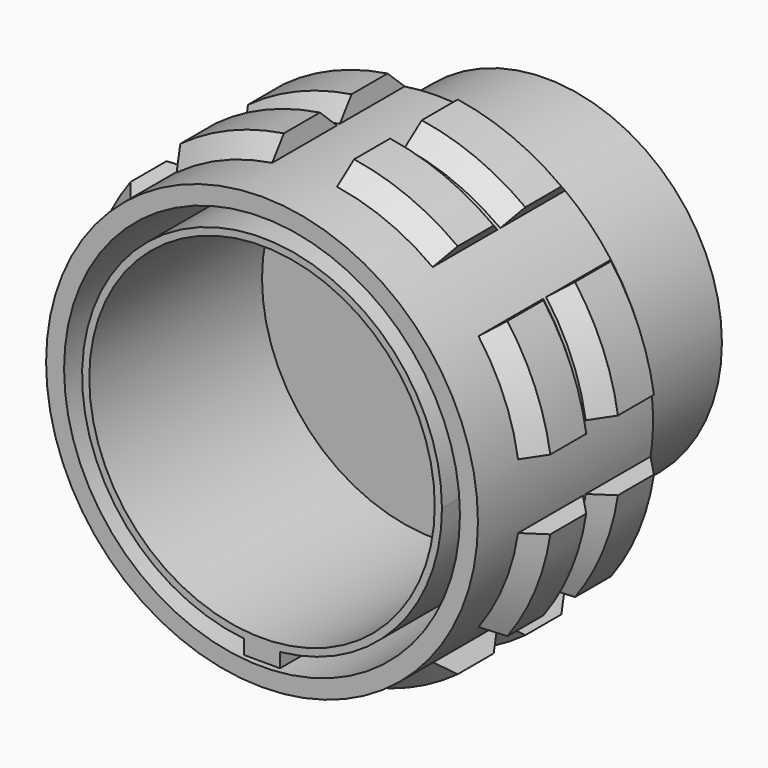
from build123d import *

# Parameters (mm, degrees)
F0_R      = 19.05
F1_DEPTH  = 15.6718
F4_DEPTH  = 14.605
F5_R      = 17.4625
F6_DEPTH  = 19.05
F7_R      = 19.05
F7_R_2    = 15.5
F8_DEPTH  = 12.0396
F10_R     = 20.6375
F10_R_2   = 19.05
F11_DEPTH = 0.15875
F12_SIZE  = 1.58749
F13_R     = 15.24
F14_DEPTH = 19.05


# Not quite as in the source:
# - a fillet or chamfer is up to 0.001 mm smaller than in the source, because OpenCascade refuses the exact size


with BuildPart() as f1:
    # F0 (on Front) → F1 (new body, symmetric)
    with BuildSketch(Plane.XZ):
        Circle(F0_R)
    extrude(amount=F1_DEPTH, both=True)

    # F3 (on offset) → F4 (join)
    with BuildSketch(Plane.XZ.offset(10.9728)):
        with BuildLine():
            Line((-20.4035253035, 3.0988), (0, 0))
            Line((0, 0), (-16.6186535957, 12.2362886087))
            ThreePointArc((-16.6186535957, 12.2362886087), (-19.0665638522, 7.8976293354), (-20.4035253035, 3.0988))
        make_face()
        with BuildLine():
            Line((-12.2362886087, 16.6186535957), (0, 0))
            Line((0, 0), (-3.0988, 20.4035253035))
            ThreePointArc((-3.0988, 20.4035253035), (-7.8976293354, 19.0665638522), (-12.2362886087, 16.6186535957))
        make_face()
        with BuildLine():
            Line((3.0988, 20.4035253035), (0, 0))
            Line((0, 0), (12.2362886087, 16.6186535957))
            ThreePointArc((12.2362886087, 16.6186535957), (7.8976293354, 19.0665638522), (3.0988, 20.4035253035))
        make_face()
        with BuildLine():
            Line((0, 0), (20.4035253035, 3.0988))
            ThreePointArc((20.4035253035, 3.0988), (19.0665638522, 7.8976293354), (16.6186535957, 12.2362886087))
            Line((16.6186535957, 12.2362886087), (0, 0))
        make_face()
        with BuildLine():
            ThreePointArc((16.6186535957, -12.2362886087), (19.0665638522, -7.8976293354), (20.4035253035, -3.0988))
            Line((20.4035253035, -3.0988), (0, 0))
            Line((0, 0), (16.6186535957, -12.2362886087))
        make_face()
        with BuildLine():
            Line((12.2362886087, -16.6186535957), (0, 0))
            Line((0, 0), (3.0988, -20.4035253035))
            ThreePointArc((3.0988, -20.4035253035), (7.8976293354, -19.0665638522), (12.2362886087, -16.6186535957))
        make_face()
        with BuildLine():
            Line((-3.0988, -20.4035253035), (0, 0))
            Line((0, 0), (-12.2362886087, -16.6186535957))
            ThreePointArc((-12.2362886087, -16.6186535957), (-7.8976293354, -19.0665638522), (-3.0988, -20.4035253035))
        make_face()
        with BuildLine():
            Line((-16.6186535957, -12.2362886087), (0, 0))
            Line((0, 0), (-20.4035253035, -3.0988))
            ThreePointArc((-20.4035253035, -3.0988), (-19.0665638522, -7.8976293354), (-16.6186535957, -12.2362886087))
        make_face()
    extrude(amount=-F4_DEPTH)

    # F5 (on face) → F6 (cut)
    with BuildSketch(Plane.XZ.offset(15.6718)):
        Circle(F5_R)
    extrude(amount=-F6_DEPTH, mode=Mode.SUBTRACT)

    # F7 (on face) → F8 (cut)
    with BuildSketch(Plane(origin=(0, 15.6718, 0), x_dir=(-1, 0, 0), z_dir=(0, 1, 0))):
        Circle(F7_R)
        Circle(F7_R_2, mode=Mode.SUBTRACT)
    extrude(amount=-F8_DEPTH, mode=Mode.SUBTRACT)

    # F10 (on offset) → F11 (cut, symmetric)
    with BuildSketch(Plane.XZ.offset(3.6703)):
        Circle(F10_R)
        Circle(F10_R_2, mode=Mode.SUBTRACT)
    extrude(amount=F11_DEPTH, both=True, mode=Mode.SUBTRACT)

    # F12 (size 1.5875 in the source; OpenCascade refuses exactly that, so slightly less here)
    f12_edges = [f1.edges().sort_by_distance(p)[0] for p in [
        (-7.897629, -3.51155, 19.066564),
        (-7.897629, -3.82905, 19.066564),
        (-7.897629, -10.9728, 19.066564),
        (-7.897629, 3.6322, 19.066564),
        (-19.066564, 3.6322, 7.897629),
        (-19.066564, -3.51155, 7.897629),
        (-19.066564, -3.82905, 7.897629),
        (-19.066564, -10.9728, 7.897629),
        (-19.066564, -10.9728, -7.897629),
        (-19.066564, -3.82905, -7.897629),
        (-19.066564, -3.51155, -7.897629),
        (-19.066564, 3.6322, -7.897629),
        (-7.897629, -10.9728, -19.066564),
        (-7.897629, -3.82905, -19.066564),
        (-7.897629, -3.51155, -19.066564),
        (-7.897629, 3.6322, -19.066564),
        (7.897629, -3.82905, -19.066564),
        (7.897629, -10.9728, -19.066564),
        (7.897629, -3.51155, -19.066564),
        (7.897629, 3.6322, -19.066564),
        (19.066564, 3.6322, -7.897629),
        (19.066564, -3.51155, -7.897629),
        (19.066564, -3.82905, -7.897629),
        (19.066564, -10.9728, -7.897629),
        (19.066564, 3.6322, 7.897629),
        (19.066564, -3.51155, 7.897629),
        (19.066564, -3.82905, 7.897629),
        (19.066564, -10.9728, 7.897629),
        (7.897629, 3.6322, 19.066564),
        (7.897629, -3.51155, 19.066564),
        (7.897629, -3.82905, 19.066564),
        (7.897629, -10.9728, 19.066564),
    ]]
    chamfer(f12_edges, length=F12_SIZE)

    # F13 (on face) → F14 (join)
    with BuildSketch(Plane.XZ.offset(-3.3782)):
        with BuildLine():
            Line((1.5875, -15.7954255641), (-1.5875, -15.7954255641))
            ThreePointArc((-1.5875, -15.7954255641), (0, -15.875), (1.5875, -15.7954255641))
        make_face()
        with BuildLine():
            ThreePointArc((1.5875, -15.7954255641), (11.7732150983, -10.6492737428), (15.875, 0))
            ThreePointArc((15.875, 0), (-10.6492737428, 11.7732150983), (-1.5875, -15.7954255641))
            Line((-1.5875, -15.7954255641), (1.5875, -15.7954255641))
        make_face()
        Circle(F13_R, mode=Mode.SUBTRACT)
        with BuildLine():
            ThreePointArc((1.5875, -15.7954255641), (0, -15.875), (-1.5875, -15.7954255641))
            Line((-1.5875, -15.7954255641), (-1.5875, -17.0654255641))
            Line((-1.5875, -17.0654255641), (1.5875, -17.0654255641))
            Line((1.5875, -17.0654255641), (1.5875, -15.7954255641))
        make_face()
    extrude(amount=F14_DEPTH)


solid = f1.part
